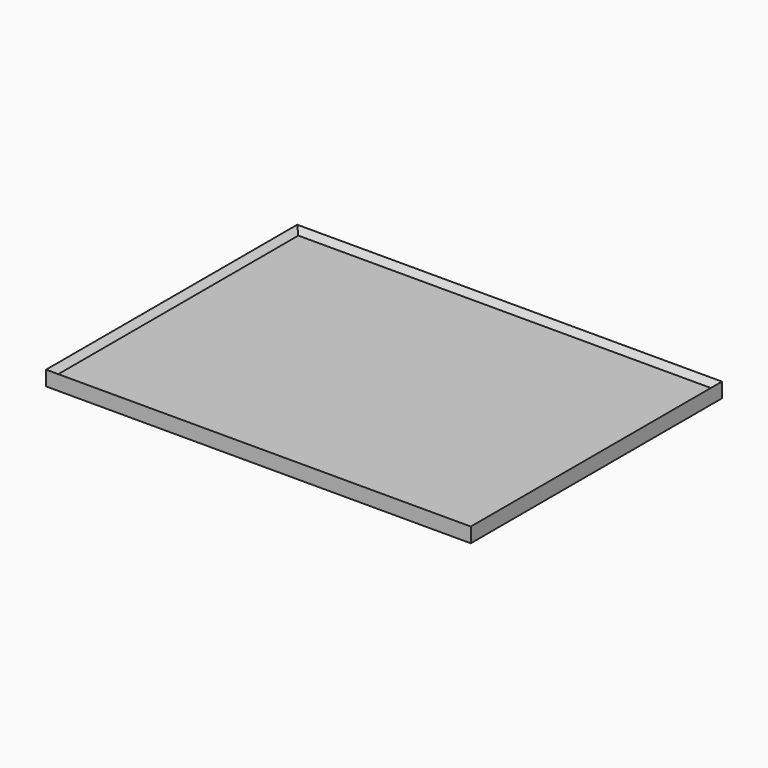
from build123d import *

# Parameters (mm, degrees)
F0_W         = 584.2
F0_H         = 431.8
F1_DEPTH     = 12.7
F2_W         = 584.2
F2_H         = 431.8
F2_W_2       = 558.8
F2_H_2       = 406.4
F3_DEPTH     = 7.62
F4_T4_DEPTH  = 558.8
F4_T9_DEPTH  = 406.4
F4_T14_DEPTH = 558.8
F4_T19_DEPTH = 406.4
F4_T25_DEPTH = 439.0603739472
F4_T31_DEPTH = 591.4603739472
F4_T40_DEPTH = 591.4603739472
F4_T46_DEPTH = 439.0603739472
F4_T55_DEPTH = 439.0603739472
F4_T61_DEPTH = 591.4603739472
F4_T70_DEPTH = 439.0603739472
F4_T76_DEPTH = 591.4603739472


# Not quite as in the source:
# - a fillet or chamfer that OpenCascade refuses, or shapes differently, is made with other operations: its cross-section is extruded or revolved along the edge and cut away or added


with BuildPart() as f1:
    # F0 (on Top) → F1 (new body)
    with BuildSketch(Plane.XY):
        Rectangle(F0_W, F0_H)
    extrude(amount=F1_DEPTH)

    # F2 (on face) → F3 (join)
    with BuildSketch(Plane.XY.offset(12.7)):
        Rectangle(F2_W, F2_H)
        Rectangle(F2_W_2, F2_H_2, mode=Mode.SUBTRACT)
    extrude(amount=F3_DEPTH)

    # F4: chamfer of 12.7 on 4 edges, made by hand


with BuildPart() as f4_tool2:
    # F4_s3 → F4_t4 (new body)
    with BuildSketch(Plane.YZ.offset(-279.4)):
        Polygon((215.9, 20.32), (203.2, 7.62), (203.2, 20.32), align=None)
    extrude(amount=F4_T4_DEPTH)

    split(bisect_by=Plane.XY.offset(12.7), keep=Keep.TOP)


with BuildPart() as f1_1:
    add(f1.part)

    # F4_t1: cut F4_tool2
    add(f4_tool2.part, mode=Mode.SUBTRACT)


with BuildPart() as f4_tool7:
    # F4_s8 → F4_t9 (new body)
    with BuildSketch(Plane.XZ.offset(-203.2)):
        Polygon((292.1, 20.32), (279.4, 7.62), (279.4, 20.32), align=None)
    extrude(amount=F4_T9_DEPTH)

    split(bisect_by=Plane.XY.offset(12.7), keep=Keep.TOP)


with BuildPart() as f1_2:
    add(f1_1.part)

    # F4_t6: cut F4_tool7
    add(f4_tool7.part, mode=Mode.SUBTRACT)


with BuildPart() as f4_tool12:
    # F4_s13 → F4_t14 (new body)
    with BuildSketch(Plane.YZ.offset(279.4)):
        Polygon((-215.9, 20.32), (-203.2, 7.62), (-203.2, 20.32), align=None)
    extrude(amount=-F4_T14_DEPTH)

    split(bisect_by=Plane.XY.offset(12.7), keep=Keep.TOP)


with BuildPart() as f1_3:
    add(f1_2.part)

    # F4_t11: cut F4_tool12
    add(f4_tool12.part, mode=Mode.SUBTRACT)


with BuildPart() as f4_tool17:
    # F4_s18 → F4_t19 (new body)
    with BuildSketch(Plane.XZ.offset(203.2)):
        Polygon((-292.1, 20.32), (-279.4, 7.62), (-279.4, 20.32), align=None)
    extrude(amount=-F4_T19_DEPTH)

    split(bisect_by=Plane.XY.offset(12.7), keep=Keep.TOP)


with BuildPart() as f1_4:
    add(f1_3.part)

    # F4_t16: cut F4_tool17
    add(f4_tool17.part, mode=Mode.SUBTRACT)


with BuildPart() as f4_tool23:
    # F4_s24 → F4_t25 (new body)
    with BuildSketch(Plane.XZ.offset(203.2)):
        Polygon((-292.1, 20.32), (-279.4, 7.62), (-279.4, 20.32), align=None)
    extrude(amount=-F4_T25_DEPTH)

    split(bisect_by=Plane.XZ.offset(-215.9), keep=Keep.TOP)

    split(bisect_by=Plane.XY.offset(12.7), keep=Keep.TOP)

    split(bisect_by=Plane.XZ.offset(-203.2), keep=Keep.BOTTOM)


with BuildPart() as f4_tool29:
    # F4_s30 → F4_t31 (new body)
    with BuildSketch(Plane.YZ.offset(-312.0603739472)):
        Polygon((215.9, 20.32), (203.2, 7.62), (203.2, 20.32), align=None)
    extrude(amount=F4_T31_DEPTH)

    split(bisect_by=Plane.XY.offset(12.7), keep=Keep.TOP)

    split(bisect_by=Plane.YZ.offset(-279.4), keep=Keep.BOTTOM)

    split(bisect_by=Plane.YZ.offset(-292.1), keep=Keep.TOP)


with BuildPart() as f4_tool23_1:
    add(f4_tool23.part)

    # F4_t35: intersect F4_tool29
    add(f4_tool29.part, mode=Mode.INTERSECT)


with BuildPart() as f1_5:
    add(f1_4.part)

    # F4_t21: cut F4_tool23
    add(f4_tool23_1.part, mode=Mode.SUBTRACT)


with BuildPart() as f4_tool38:
    # F4_s39 → F4_t40 (new body)
    with BuildSketch(Plane.YZ.offset(-279.4)):
        Polygon((215.9, 20.32), (203.2, 7.62), (203.2, 20.32), align=None)
    extrude(amount=F4_T40_DEPTH)

    split(bisect_by=Plane.YZ.offset(292.1), keep=Keep.BOTTOM)

    split(bisect_by=Plane.XY.offset(12.7), keep=Keep.TOP)

    split(bisect_by=Plane.YZ.offset(279.4), keep=Keep.TOP)


with BuildPart() as f4_tool44:
    # F4_s45 → F4_t46 (new body)
    with BuildSketch(Plane.XZ.offset(-235.8603739472)):
        Polygon((292.1, 20.32), (279.4, 7.62), (279.4, 20.32), align=None)
    extrude(amount=F4_T46_DEPTH)

    split(bisect_by=Plane.XZ.offset(-215.9), keep=Keep.TOP)

    split(bisect_by=Plane.XY.offset(12.7), keep=Keep.TOP)

    split(bisect_by=Plane.XZ.offset(-203.2), keep=Keep.BOTTOM)


with BuildPart() as f4_tool38_1:
    add(f4_tool38.part)

    # F4_t50: intersect F4_tool44
    add(f4_tool44.part, mode=Mode.INTERSECT)


with BuildPart() as f1_6:
    add(f1_5.part)

    # F4_t36: cut F4_tool38
    add(f4_tool38_1.part, mode=Mode.SUBTRACT)


with BuildPart() as f4_tool53:
    # F4_s54 → F4_t55 (new body)
    with BuildSketch(Plane.XZ.offset(-203.2)):
        Polygon((292.1, 20.32), (279.4, 7.62), (279.4, 20.32), align=None)
    extrude(amount=F4_T55_DEPTH)

    split(bisect_by=Plane.XZ.offset(215.9), keep=Keep.BOTTOM)

    split(bisect_by=Plane.XZ.offset(203.2), keep=Keep.TOP)

    split(bisect_by=Plane.XY.offset(12.7), keep=Keep.TOP)


with BuildPart() as f4_tool59:
    # F4_s60 → F4_t61 (new body)
    with BuildSketch(Plane.YZ.offset(312.0603739472)):
        Polygon((-215.9, 20.32), (-203.2, 7.62), (-203.2, 20.32), align=None)
    extrude(amount=-F4_T61_DEPTH)

    split(bisect_by=Plane.YZ.offset(292.1), keep=Keep.BOTTOM)

    split(bisect_by=Plane.XY.offset(12.7), keep=Keep.TOP)

    split(bisect_by=Plane.YZ.offset(279.4), keep=Keep.TOP)


with BuildPart() as f4_tool53_1:
    add(f4_tool53.part)

    # F4_t65: intersect F4_tool59
    add(f4_tool59.part, mode=Mode.INTERSECT)


with BuildPart() as f1_7:
    add(f1_6.part)

    # F4_t51: cut F4_tool53
    add(f4_tool53_1.part, mode=Mode.SUBTRACT)


with BuildPart() as f4_tool68:
    # F4_s69 → F4_t70 (new body)
    with BuildSketch(Plane.XZ.offset(235.8603739472)):
        Polygon((-292.1, 20.32), (-279.4, 7.62), (-279.4, 20.32), align=None)
    extrude(amount=-F4_T70_DEPTH)

    split(bisect_by=Plane.XZ.offset(215.9), keep=Keep.BOTTOM)

    split(bisect_by=Plane.XZ.offset(203.2), keep=Keep.TOP)

    split(bisect_by=Plane.XY.offset(12.7), keep=Keep.TOP)


with BuildPart() as f4_tool74:
    # F4_s75 → F4_t76 (new body)
    with BuildSketch(Plane.YZ.offset(279.4)):
        Polygon((-215.9, 20.32), (-203.2, 7.62), (-203.2, 20.32), align=None)
    extrude(amount=-F4_T76_DEPTH)

    split(bisect_by=Plane.XY.offset(12.7), keep=Keep.TOP)

    split(bisect_by=Plane.YZ.offset(-279.4), keep=Keep.BOTTOM)

    split(bisect_by=Plane.YZ.offset(-292.1), keep=Keep.TOP)


with BuildPart() as f4_tool68_1:
    add(f4_tool68.part)

    # F4_t80: intersect F4_tool74
    add(f4_tool74.part, mode=Mode.INTERSECT)


with BuildPart() as f1_8:
    add(f1_7.part)

    # F4_t66: cut F4_tool68
    add(f4_tool68_1.part, mode=Mode.SUBTRACT)


solid = f1_8.part
